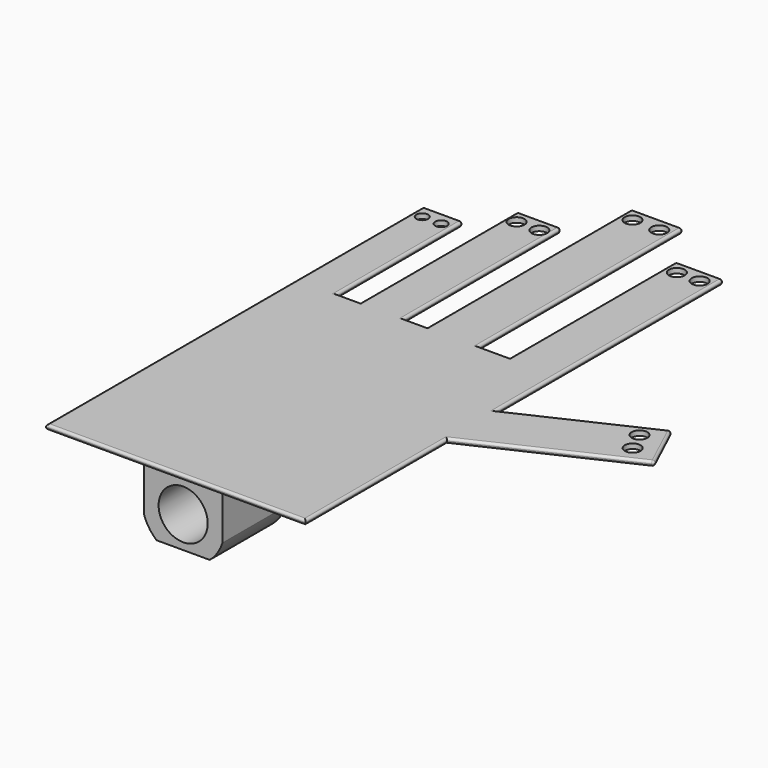
from build123d import *

# Parameters (mm, degrees)
F0_W          = 12.7
F0_H          = 50.8
F0_W_2        = 13.97
F0_H_2        = 63.5
F0_W_3        = 16.51
F0_H_3        = 82.55
F0_W_4        = 15.24
F0_H_4        = 67.123832345
F1_DEPTH      = 1.5875
F2_R          = 0.762
F3_R          = 0.762
F4_T1_DEPTH   = 87.63
F4_T3_DEPTH   = 153.543
F4_T5_DEPTH   = 66.361832345
F4_T7_DEPTH   = 50.038
F4_T9_DEPTH   = 10.16
F4_T11_DEPTH  = 7.62
F4_T13_DEPTH  = 81.788
F4_T15_DEPTH  = 62.738
F4_T17_DEPTH  = 7.62
F4_T19_DEPTH  = 0.0635
F4_T24_DEPTH  = 55.0115454207
F4_T29_DEPTH  = 61.0436683929
F4_T34_DEPTH  = 46.7205952588
F4_T39_DEPTH  = 93.015104553
F4_T44_DEPTH  = 55.0115454207
F4_T49_DEPTH  = 61.0436683929
F4_T54_DEPTH  = 46.7205952588
F4_T59_DEPTH  = 93.015104553
F4_T62_ANGLE  = 90
F4_T64_ANGLE  = 90
F4_T66_ANGLE  = 90
F4_T68_ANGLE  = 90
F4_T70_ANGLE  = 90
F4_T72_ANGLE  = 90
F4_T74_ANGLE  = 90
F4_T76_ANGLE  = 90
F4_T78_ANGLE  = 90
F4_T80_ANGLE  = 90
F4_T82_ANGLE  = 90
F4_T84_ANGLE  = 90
F4_T86_ANGLE  = 90
F4_T88_ANGLE  = 90
F4_T90_ANGLE  = 90
F4_T92_ANGLE  = 90
F4_T94_ANGLE  = 90
F4_T96_ANGLE  = 90
F4_T98_ANGLE  = 90
F4_T100_ANGLE = 90
F4_T105_DEPTH = 55.0115454207
F4_T109_DEPTH = 61.0436683929
F4_T116_DEPTH = 46.7205952588
F4_T120_DEPTH = 93.015104553
F4_T127_DEPTH = 68.266832345
F4_T131_DEPTH = 12.065
F4_T138_DEPTH = 51.943
F4_T142_DEPTH = 9.525
F4_T149_DEPTH = 12.065
F4_T153_DEPTH = 83.693
F4_T160_DEPTH = 9.525
F4_T164_DEPTH = 64.643
F4_T171_DEPTH = 83.693
F4_T175_DEPTH = 9.525
F4_T182_DEPTH = 64.643
F4_T186_DEPTH = 9.525
F4_T193_DEPTH = 55.0115454207
F4_T197_DEPTH = 61.0436683929
F4_T204_DEPTH = 46.7205952588
F4_T208_DEPTH = 93.015104553
F4_T215_DEPTH = 68.266832345
F4_T219_DEPTH = 12.065
F4_T226_DEPTH = 51.943
F4_T230_DEPTH = 9.525
F4_T237_DEPTH = 12.065
F4_T241_DEPTH = 83.693
F4_T248_DEPTH = 9.525
F4_T252_DEPTH = 64.643
F4_T259_DEPTH = 83.693
F4_T263_DEPTH = 9.525
F4_T270_DEPTH = 64.643
F4_T274_DEPTH = 9.525
F5_R          = 2.54
F5_R_2        = 1.905
F6_DEPTH      = 25.4
F7_W          = 25.4
F7_H          = 25.4
F8_DEPTH      = 20.32
F9_R          = 7.9375
F10_DEPTH     = 25.4
F12_DEPTH     = 25.4


# Not quite as in the source:
# - a fillet or chamfer that OpenCascade refuses, or shapes differently, is made with other operations: its cross-section is extruded or revolved along the edge and cut away or added


with BuildPart() as f1:
    # F0 (on Top) → F1 (new body)
    with BuildSketch(Plane.XY):
        Polygon((-47.5871736486, 71.2477097511), (-47.5871736486, -30.3522902489), (36.2328263514, -30.3522902489), (36.2328263514, 26.881378144), (36.2328263514, 46.4994375432), (36.2328263514, 71.2477097511), (20.9928263514, 71.2477097511), (10.8328263514, 71.2477097511), (-5.6771736486, 71.2477097511), (-13.2971736486, 71.2477097511), (-27.2671736486, 71.2477097511), (-34.8871736486, 71.2477097511), align=None)
        with Locations((-41.2371736486, 96.6477097511)):
            Rectangle(F0_W, F0_H)
        with Locations((-20.2821736486, 102.9977097511)):
            Rectangle(F0_W_2, F0_H_2)
        with Locations((2.5778263514, 112.5227097511)):
            Rectangle(F0_W_3, F0_H_3)
        with Locations((28.6128263514, 104.8096259236)):
            Rectangle(F0_W_4, F0_H_4)
        Polygon((36.2328263514, 46.4994375432), (36.2328263514, 26.881378144), (85.0543085426, 49.6472091722), (77.5401558489, 65.7613616258), align=None)
    extrude(amount=F1_DEPTH)

    # F2
    f2_edges = [f1.edges().sort_by_distance(p)[0] for p in [
        (-41.237174, 122.04771, 1.5875),
        (-20.282174, 134.74771, 1.5875),
        (2.577826, 153.79771, 1.5875),
        (28.612826, 138.371542, 1.5875),
        (81.297232, 57.704285, 1.5875),
    ]]
    fillet(f2_edges, radius=F2_R)

    # F3
    f3_edges = [f1.edges().sort_by_distance(p)[0] for p in [
        (81.297232, 57.704285, 0),
        (28.612826, 138.371542, 0),
        (2.577826, 153.79771, 0),
        (-20.282174, 134.74771, 0),
        (-41.237174, 122.04771, 0),
    ]]
    fillet(f3_edges, radius=F3_R)

    # F4: fillet of radius 0.762 on 70 edges, made by hand

    # F4_s2 → F4_t1 (cut)
    with BuildSketch(Plane.YZ.offset(-49.4921736486)):
        with BuildLine():
            ThreePointArc((-29.5902902489, 1.5875), (-30.1291056161, 1.3643153673), (-30.3522902489, 0.8255))
            Line((-30.3522902489, 0.8255), (-30.3522902489, 1.5875))
            Line((-30.3522902489, 1.5875), (-29.5902902489, 1.5875))
        make_face()
        with BuildLine():
            ThreePointArc((-29.5902902489, 0), (-30.1291056161, 0.2231846327), (-30.3522902489, 0.762))
            Line((-30.3522902489, 0.762), (-30.3522902489, 0))
            Line((-30.3522902489, 0), (-29.5902902489, 0))
        make_face()
    extrude(amount=F4_T1_DEPTH, mode=Mode.SUBTRACT)

    # F4_s4 → F4_t3 (cut)
    with BuildSketch(Plane.XZ.offset(-121.2857097511)):
        with BuildLine():
            ThreePointArc((-46.8251736486, 1.5875), (-47.3639890158, 1.3643153673), (-47.5871736486, 0.8255))
            Line((-47.5871736486, 0.8255), (-47.5871736486, 1.5875))
            Line((-47.5871736486, 1.5875), (-46.8251736486, 1.5875))
        make_face()
        with BuildLine():
            ThreePointArc((-46.8251736486, 0), (-47.3639890158, 0.2231846327), (-47.5871736486, 0.762))
            Line((-47.5871736486, 0.762), (-47.5871736486, 0))
            Line((-47.5871736486, 0), (-46.8251736486, 0))
        make_face()
    extrude(amount=F4_T3_DEPTH, mode=Mode.SUBTRACT)

    # F4_s6 → F4_t5 (cut)
    with BuildSketch(Plane.XZ.offset(-137.6095420961)):
        with BuildLine():
            ThreePointArc((21.7548263514, 1.5875), (21.2160109842, 1.3643153673), (20.9928263514, 0.8255))
            Line((20.9928263514, 0.8255), (20.9928263514, 1.5875))
            Line((20.9928263514, 1.5875), (21.7548263514, 1.5875))
        make_face()
        with BuildLine():
            ThreePointArc((21.7548263514, 0), (21.2160109842, 0.2231846327), (20.9928263514, 0.762))
            Line((20.9928263514, 0.762), (20.9928263514, 0))
            Line((20.9928263514, 0), (21.7548263514, 0))
        make_face()
    extrude(amount=F4_T5_DEPTH, mode=Mode.SUBTRACT)

    # F4_s8 → F4_t7 (cut)
    with BuildSketch(Plane.XZ.offset(-121.2857097511)):
        with BuildLine():
            ThreePointArc((-35.6491736486, 1.5875), (-35.1103582813, 1.3643153673), (-34.8871736486, 0.8255))
            Line((-34.8871736486, 0.8255), (-34.8871736486, 1.5875))
            Line((-34.8871736486, 1.5875), (-35.6491736486, 1.5875))
        make_face()
        with BuildLine():
            ThreePointArc((-35.6491736486, 0), (-35.1103582813, 0.2231846327), (-34.8871736486, 0.762))
            Line((-34.8871736486, 0.762), (-34.8871736486, 0))
            Line((-34.8871736486, 0), (-35.6491736486, 0))
        make_face()
    extrude(amount=F4_T7_DEPTH, mode=Mode.SUBTRACT)

    # F4_s10 → F4_t9 (cut)
    with BuildSketch(Plane.YZ.offset(10.8328263514)):
        with BuildLine():
            ThreePointArc((70.4857097511, 1.5875), (71.0245251184, 1.3643153673), (71.2477097511, 0.8255))
            Line((71.2477097511, 0.8255), (71.2477097511, 1.5875))
            Line((71.2477097511, 1.5875), (70.4857097511, 1.5875))
        make_face()
        with BuildLine():
            ThreePointArc((70.4857097511, 0), (71.0245251184, 0.2231846327), (71.2477097511, 0.762))
            Line((71.2477097511, 0.762), (71.2477097511, 0))
            Line((71.2477097511, 0), (70.4857097511, 0))
        make_face()
    extrude(amount=F4_T9_DEPTH, mode=Mode.SUBTRACT)

    # F4_s12 → F4_t11 (cut)
    with BuildSketch(Plane.YZ.offset(-34.8871736486)):
        with BuildLine():
            ThreePointArc((70.4857097511, 1.5875), (71.0245251184, 1.3643153673), (71.2477097511, 0.8255))
            Line((71.2477097511, 0.8255), (71.2477097511, 1.5875))
            Line((71.2477097511, 1.5875), (70.4857097511, 1.5875))
        make_face()
        with BuildLine():
            ThreePointArc((70.4857097511, 0), (71.0245251184, 0.2231846327), (71.2477097511, 0.762))
            Line((71.2477097511, 0.762), (71.2477097511, 0))
            Line((71.2477097511, 0), (70.4857097511, 0))
        make_face()
    extrude(amount=F4_T11_DEPTH, mode=Mode.SUBTRACT)

    # F4_s14 → F4_t13 (cut)
    with BuildSketch(Plane.XZ.offset(-153.0357097511)):
        with BuildLine():
            ThreePointArc((10.0708263514, 1.5875), (10.6096417187, 1.3643153673), (10.8328263514, 0.8255))
            Line((10.8328263514, 0.8255), (10.8328263514, 1.5875))
            Line((10.8328263514, 1.5875), (10.0708263514, 1.5875))
        make_face()
        with BuildLine():
            ThreePointArc((-4.9151736486, 1.5875), (-5.4539890158, 1.3643153673), (-5.6771736486, 0.8255))
            Line((-5.6771736486, 0.8255), (-5.6771736486, 1.5875))
            Line((-5.6771736486, 1.5875), (-4.9151736486, 1.5875))
        make_face()
        with BuildLine():
            ThreePointArc((10.0708263514, 0), (10.6096417187, 0.2231846327), (10.8328263514, 0.762))
            Line((10.8328263514, 0.762), (10.8328263514, 0))
            Line((10.8328263514, 0), (10.0708263514, 0))
        make_face()
        with BuildLine():
            ThreePointArc((-4.9151736486, 0), (-5.4539890158, 0.2231846327), (-5.6771736486, 0.762))
            Line((-5.6771736486, 0.762), (-5.6771736486, 0))
            Line((-5.6771736486, 0), (-4.9151736486, 0))
        make_face()
    extrude(amount=F4_T13_DEPTH, mode=Mode.SUBTRACT)

    # F4_s16 → F4_t15 (cut)
    with BuildSketch(Plane.XZ.offset(-133.9857097511)):
        with BuildLine():
            ThreePointArc((-26.5051736486, 1.5875), (-27.0439890158, 1.3643153673), (-27.2671736486, 0.8255))
            Line((-27.2671736486, 0.8255), (-27.2671736486, 1.5875))
            Line((-27.2671736486, 1.5875), (-26.5051736486, 1.5875))
        make_face()
        with BuildLine():
            ThreePointArc((-14.0591736486, 1.5875), (-13.5203582813, 1.3643153673), (-13.2971736486, 0.8255))
            Line((-13.2971736486, 0.8255), (-13.2971736486, 1.5875))
            Line((-13.2971736486, 1.5875), (-14.0591736486, 1.5875))
        make_face()
        with BuildLine():
            ThreePointArc((-26.5051736486, 0), (-27.0439890158, 0.2231846327), (-27.2671736486, 0.762))
            Line((-27.2671736486, 0.762), (-27.2671736486, 0))
            Line((-27.2671736486, 0), (-26.5051736486, 0))
        make_face()
        with BuildLine():
            ThreePointArc((-14.0591736486, 0), (-13.5203582813, 0.2231846327), (-13.2971736486, 0.762))
            Line((-13.2971736486, 0.762), (-13.2971736486, 0))
            Line((-13.2971736486, 0), (-14.0591736486, 0))
        make_face()
    extrude(amount=F4_T15_DEPTH, mode=Mode.SUBTRACT)

    # F4_s18 → F4_t17 (cut)
    with BuildSketch(Plane.YZ.offset(-13.2971736486)):
        with BuildLine():
            ThreePointArc((70.4857097511, 1.5875), (71.0245251184, 1.3643153673), (71.2477097511, 0.8255))
            Line((71.2477097511, 0.8255), (71.2477097511, 1.5875))
            Line((71.2477097511, 1.5875), (70.4857097511, 1.5875))
        make_face()
        with BuildLine():
            ThreePointArc((70.4857097511, 0), (71.0245251184, 0.2231846327), (71.2477097511, 0.762))
            Line((71.2477097511, 0.762), (71.2477097511, 0))
            Line((71.2477097511, 0), (70.4857097511, 0))
        make_face()
    extrude(amount=F4_T17_DEPTH, mode=Mode.SUBTRACT)

    # F4_s20 → F4_t19 (cut)
    with BuildSketch(Plane.XY.offset(0.762)):
        with BuildLine():
            ThreePointArc((84.3637020089, 49.3251740568), (84.7577126705, 49.7551612413), (84.7322734272, 50.337815706))
            Line((84.7322734272, 50.337815706), (85.0543085426, 49.6472091722))
            Line((85.0543085426, 49.6472091722), (84.3637020089, 49.3251740568))
        make_face()
        with BuildLine():
            ThreePointArc((77.8621909643, 65.070755092), (77.4322037798, 65.4647657536), (76.8495493151, 65.4393265103))
            Line((76.8495493151, 65.4393265103), (77.5401558489, 65.7613616258))
            Line((77.5401558489, 65.7613616258), (77.8621909643, 65.070755092))
        make_face()
        with BuildLine():
            ThreePointArc((36.2328263514, 137.6095420961), (36.0096417187, 138.1483574634), (35.4708263514, 138.3715420961))
            Line((35.4708263514, 138.3715420961), (36.2328263514, 138.3715420961))
            Line((36.2328263514, 138.3715420961), (36.2328263514, 137.6095420961))
        make_face()
        with BuildLine():
            ThreePointArc((-47.5871736486, 121.2857097511), (-47.3639890158, 121.8245251184), (-46.8251736486, 122.0477097511))
            Line((-46.8251736486, 122.0477097511), (-47.5871736486, 122.0477097511))
            Line((-47.5871736486, 122.0477097511), (-47.5871736486, 121.2857097511))
        make_face()
        with BuildLine():
            ThreePointArc((20.9928263514, 137.6095420961), (21.2160109842, 138.1483574634), (21.7548263514, 138.3715420961))
            Line((21.7548263514, 138.3715420961), (20.9928263514, 138.3715420961))
            Line((20.9928263514, 138.3715420961), (20.9928263514, 137.6095420961))
        make_face()
        with BuildLine():
            ThreePointArc((-34.8871736486, 121.2857097511), (-35.1103582813, 121.8245251184), (-35.6491736486, 122.0477097511))
            Line((-35.6491736486, 122.0477097511), (-34.8871736486, 122.0477097511))
            Line((-34.8871736486, 122.0477097511), (-34.8871736486, 121.2857097511))
        make_face()
        with BuildLine():
            ThreePointArc((10.8328263514, 153.0357097511), (10.6096417187, 153.5745251184), (10.0708263514, 153.7977097511))
            Line((10.0708263514, 153.7977097511), (10.8328263514, 153.7977097511))
            Line((10.8328263514, 153.7977097511), (10.8328263514, 153.0357097511))
        make_face()
        with BuildLine():
            ThreePointArc((-27.2671736486, 133.9857097511), (-27.0439890158, 134.5245251184), (-26.5051736486, 134.7477097511))
            Line((-26.5051736486, 134.7477097511), (-27.2671736486, 134.7477097511))
            Line((-27.2671736486, 134.7477097511), (-27.2671736486, 133.9857097511))
        make_face()
        with BuildLine():
            ThreePointArc((-5.6771736486, 153.0357097511), (-5.4539890158, 153.5745251184), (-4.9151736486, 153.7977097511))
            Line((-4.9151736486, 153.7977097511), (-5.6771736486, 153.7977097511))
            Line((-5.6771736486, 153.7977097511), (-5.6771736486, 153.0357097511))
        make_face()
        with BuildLine():
            ThreePointArc((-13.2971736486, 133.9857097511), (-13.5203582813, 134.5245251184), (-14.0591736486, 134.7477097511))
            Line((-14.0591736486, 134.7477097511), (-13.2971736486, 134.7477097511))
            Line((-13.2971736486, 134.7477097511), (-13.2971736486, 133.9857097511))
        make_face()
    extrude(amount=F4_T19_DEPTH, mode=Mode.SUBTRACT)


with BuildPart() as f4_tool22:
    # F4_s23 → F4_t24 (new body)
    with BuildSketch(Plane(origin=(38.331067938, 17.8740705248, 0), x_dir=(0, 0, 1), z_dir=(0.906307787, 0.4226182617, 0))):
        with BuildLine():
            ThreePointArc((0.8255, -9.0501482476), (1.3643153673, -9.2733328803), (1.5875, -9.8121482476))
            Line((1.5875, -9.8121482476), (1.5875, -9.0501482476))
            Line((1.5875, -9.0501482476), (0.8255, -9.0501482476))
        make_face()
    extrude(amount=F4_T24_DEPTH)

    split(bisect_by=Plane.YZ.offset(36.2328263514), keep=Keep.TOP)


with BuildPart() as f1_1:
    add(f1.part)

    # F4_t21: cut F4_tool22
    add(f4_tool22.part, mode=Mode.SUBTRACT)


with BuildPart() as f4_tool27:
    # F4_s28 → F4_t29 (new body)
    with BuildSketch(Plane.XZ.offset(32.2572902489)):
        with BuildLine():
            ThreePointArc((35.4708263514, 1.5875), (36.0096417187, 1.3643153673), (36.2328263514, 0.8255))
            Line((36.2328263514, 0.8255), (36.2328263514, 1.5875))
            Line((36.2328263514, 1.5875), (35.4708263514, 1.5875))
        make_face()
    extrude(amount=-F4_T29_DEPTH)

    split(bisect_by=Plane(origin=(-3.8247579209, 8.2022198306, 0), x_dir=(0, 0, 1), z_dir=(0.4226182617, -0.906307787, 0)), keep=Keep.TOP)


with BuildPart() as f1_2:
    add(f1_1.part)

    # F4_t26: cut F4_tool27
    add(f4_tool27.part, mode=Mode.SUBTRACT)


with BuildPart() as f4_tool32:
    # F4_s33 → F4_t34 (new body)
    with BuildSketch(Plane(origin=(88.1884599298, 41.1229542262, 0), x_dir=(0, 0, 1), z_dir=(-0.906307787, -0.4226182617, 0))):
        with BuildLine():
            ThreePointArc((1.5875, 26.0681482476), (1.3643153673, 26.6069636149), (0.8255, 26.8301482476))
            Line((0.8255, 26.8301482476), (1.5875, 26.8301482476))
            Line((1.5875, 26.8301482476), (1.5875, 26.0681482476))
        make_face()
    extrude(amount=F4_T34_DEPTH)

    split(bisect_by=Plane.YZ.offset(36.2328263514), keep=Keep.TOP)


with BuildPart() as f1_3:
    add(f1_2.part)

    # F4_t31: cut F4_tool32
    add(f4_tool32.part, mode=Mode.SUBTRACT)


with BuildPart() as f4_tool37:
    # F4_s38 → F4_t39 (new body)
    with BuildSketch(Plane.XZ.offset(-44.5944375432)):
        with BuildLine():
            ThreePointArc((35.4708263514, 1.5875), (36.0096417187, 1.3643153673), (36.2328263514, 0.8255))
            Line((36.2328263514, 0.8255), (36.2328263514, 1.5875))
            Line((36.2328263514, 1.5875), (35.4708263514, 1.5875))
        make_face()
    extrude(amount=-F4_T39_DEPTH)

    split(bisect_by=Plane(origin=(-11.3389106146, 24.3163722842, 0), x_dir=(0, 0, 1), z_dir=(-0.4226182617, 0.906307787, 0)), keep=Keep.TOP)


with BuildPart() as f1_4:
    add(f1_3.part)

    # F4_t36: cut F4_tool37
    add(f4_tool37.part, mode=Mode.SUBTRACT)


with BuildPart() as f4_tool42:
    # F4_s43 → F4_t44 (new body)
    with BuildSketch(Plane(origin=(38.331067938, 17.8740705248, 0), x_dir=(0, 0, 1), z_dir=(0.906307787, 0.4226182617, 0))):
        with BuildLine():
            ThreePointArc((0.762, -9.0501482476), (0.2231846327, -9.2733328803), (0, -9.8121482476))
            Line((0, -9.8121482476), (0, -9.0501482476))
            Line((0, -9.0501482476), (0.762, -9.0501482476))
        make_face()
    extrude(amount=F4_T44_DEPTH)

    split(bisect_by=Plane.YZ.offset(36.2328263514), keep=Keep.TOP)


with BuildPart() as f1_5:
    add(f1_4.part)

    # F4_t41: cut F4_tool42
    add(f4_tool42.part, mode=Mode.SUBTRACT)


with BuildPart() as f4_tool47:
    # F4_s48 → F4_t49 (new body)
    with BuildSketch(Plane.XZ.offset(32.2572902489)):
        with BuildLine():
            ThreePointArc((35.4708263514, 0), (36.0096417187, 0.2231846327), (36.2328263514, 0.762))
            Line((36.2328263514, 0.762), (36.2328263514, 0))
            Line((36.2328263514, 0), (35.4708263514, 0))
        make_face()
    extrude(amount=-F4_T49_DEPTH)

    split(bisect_by=Plane(origin=(-3.8247579209, 8.2022198306, 0), x_dir=(0, 0, 1), z_dir=(0.4226182617, -0.906307787, 0)), keep=Keep.TOP)


with BuildPart() as f1_6:
    add(f1_5.part)

    # F4_t46: cut F4_tool47
    add(f4_tool47.part, mode=Mode.SUBTRACT)


with BuildPart() as f4_tool52:
    # F4_s53 → F4_t54 (new body)
    with BuildSketch(Plane(origin=(88.1884599298, 41.1229542262, 0), x_dir=(0, 0, 1), z_dir=(-0.906307787, -0.4226182617, 0))):
        with BuildLine():
            ThreePointArc((0, 26.0681482476), (0.2231846327, 26.6069636149), (0.762, 26.8301482476))
            Line((0.762, 26.8301482476), (0, 26.8301482476))
            Line((0, 26.8301482476), (0, 26.0681482476))
        make_face()
    extrude(amount=F4_T54_DEPTH)

    split(bisect_by=Plane.YZ.offset(36.2328263514), keep=Keep.TOP)


with BuildPart() as f1_7:
    add(f1_6.part)

    # F4_t51: cut F4_tool52
    add(f4_tool52.part, mode=Mode.SUBTRACT)


with BuildPart() as f4_tool57:
    # F4_s58 → F4_t59 (new body)
    with BuildSketch(Plane.XZ.offset(-44.5944375432)):
        with BuildLine():
            ThreePointArc((35.4708263514, 0), (36.0096417187, 0.2231846327), (36.2328263514, 0.762))
            Line((36.2328263514, 0.762), (36.2328263514, 0))
            Line((36.2328263514, 0), (35.4708263514, 0))
        make_face()
    extrude(amount=-F4_T59_DEPTH)

    split(bisect_by=Plane(origin=(-11.3389106146, 24.3163722842, 0), x_dir=(0, 0, 1), z_dir=(-0.4226182617, 0.906307787, 0)), keep=Keep.TOP)


with BuildPart() as f1_8:
    add(f1_7.part)

    # F4_t56: cut F4_tool57
    add(f4_tool57.part, mode=Mode.SUBTRACT)

    # F4_s61 → F4_t62 (revolve, cut)
    with BuildSketch(Plane.XY.offset(0.762)):
        with BuildLine():
            ThreePointArc((84.3637020089, 49.3251740568), (84.7577126705, 49.7551612413), (84.7322734272, 50.337815706))
            Line((84.7322734272, 50.337815706), (85.0543085426, 49.6472091722))
            Line((85.0543085426, 49.6472091722), (84.3637020089, 49.3251740568))
        make_face()
    revolve(axis=Axis((84.3637020089, 49.3251740568, 0.762), (-0.4226182617, 0.906307787, 0)), revolution_arc=F4_T62_ANGLE, mode=Mode.SUBTRACT)

    # F4_s63 → F4_t64 (revolve, cut)
    with BuildSketch(Plane.XY.offset(0.8255)):
        with BuildLine():
            ThreePointArc((84.3637020089, 49.3251740568), (84.7577126705, 49.7551612413), (84.7322734272, 50.337815706))
            Line((84.7322734272, 50.337815706), (85.0543085426, 49.6472091722))
            Line((85.0543085426, 49.6472091722), (84.3637020089, 49.3251740568))
        make_face()
    revolve(axis=Axis((84.3637020089, 49.3251740568, 0.8255), (0.4226182617, -0.906307787, 0)), revolution_arc=F4_T64_ANGLE, mode=Mode.SUBTRACT)

    # F4_s65 → F4_t66 (revolve, cut)
    with BuildSketch(Plane.XY.offset(0.762)):
        with BuildLine():
            ThreePointArc((77.8621909643, 65.070755092), (77.4322037798, 65.4647657536), (76.8495493151, 65.4393265103))
            Line((76.8495493151, 65.4393265103), (77.5401558489, 65.7613616258))
            Line((77.5401558489, 65.7613616258), (77.8621909643, 65.070755092))
        make_face()
    revolve(axis=Axis((76.8495493151, 65.4393265103, 0.762), (-0.4226182617, 0.906307787, 0)), revolution_arc=F4_T66_ANGLE, mode=Mode.SUBTRACT)

    # F4_s67 → F4_t68 (revolve, cut)
    with BuildSketch(Plane.XY.offset(0.8255)):
        with BuildLine():
            ThreePointArc((77.8621909643, 65.070755092), (77.4322037798, 65.4647657536), (76.8495493151, 65.4393265103))
            Line((76.8495493151, 65.4393265103), (77.5401558489, 65.7613616258))
            Line((77.5401558489, 65.7613616258), (77.8621909643, 65.070755092))
        make_face()
    revolve(axis=Axis((76.8495493151, 65.4393265103, 0.8255), (0.4226182617, -0.906307787, 0)), revolution_arc=F4_T68_ANGLE, mode=Mode.SUBTRACT)

    # F4_s69 → F4_t70 (revolve, cut)
    with BuildSketch(Plane.XZ.offset(-137.6095420961)):
        with BuildLine():
            ThreePointArc((36.2328263514, 0.762), (36.0096417187, 0.2231846327), (35.4708263514, 0))
            Line((35.4708263514, 0), (36.2328263514, 0))
            Line((36.2328263514, 0), (36.2328263514, 0.762))
        make_face()
    revolve(axis=Axis((36.2328263514, 137.6095420961, 0.762), (1, 0, 0)), revolution_arc=F4_T70_ANGLE, mode=Mode.SUBTRACT)

    # F4_s71 → F4_t72 (revolve, cut)
    with BuildSketch(Plane.XY.offset(0.8255)):
        with BuildLine():
            ThreePointArc((36.2328263514, 137.6095420961), (36.0096417187, 138.1483574634), (35.4708263514, 138.3715420961))
            Line((35.4708263514, 138.3715420961), (36.2328263514, 138.3715420961))
            Line((36.2328263514, 138.3715420961), (36.2328263514, 137.6095420961))
        make_face()
    revolve(axis=Axis((36.2328263514, 137.6095420961, 0.8255), (1, 0, 0)), revolution_arc=F4_T72_ANGLE, mode=Mode.SUBTRACT)

    # F4_s73 → F4_t74 (revolve, cut)
    with BuildSketch(Plane.XZ.offset(-121.2857097511)):
        with BuildLine():
            ThreePointArc((-47.5871736486, 0.762), (-47.3639890158, 0.2231846327), (-46.8251736486, 0))
            Line((-46.8251736486, 0), (-47.5871736486, 0))
            Line((-47.5871736486, 0), (-47.5871736486, 0.762))
        make_face()
    revolve(axis=Axis((-47.5871736486, 121.2857097511, 0.762), (1, 0, 0)), revolution_arc=F4_T74_ANGLE, mode=Mode.SUBTRACT)

    # F4_s75 → F4_t76 (revolve, cut)
    with BuildSketch(Plane.XY.offset(0.8255)):
        with BuildLine():
            ThreePointArc((-47.5871736486, 121.2857097511), (-47.3639890158, 121.8245251184), (-46.8251736486, 122.0477097511))
            Line((-46.8251736486, 122.0477097511), (-47.5871736486, 122.0477097511))
            Line((-47.5871736486, 122.0477097511), (-47.5871736486, 121.2857097511))
        make_face()
    revolve(axis=Axis((-47.5871736486, 121.2857097511, 0.8255), (1, 0, 0)), revolution_arc=F4_T76_ANGLE, mode=Mode.SUBTRACT)

    # F4_s77 → F4_t78 (revolve, cut)
    with BuildSketch(Plane.XZ.offset(-137.6095420961)):
        with BuildLine():
            ThreePointArc((21.7548263514, 0), (21.2160109842, 0.2231846327), (20.9928263514, 0.762))
            Line((20.9928263514, 0.762), (20.9928263514, 0))
            Line((20.9928263514, 0), (21.7548263514, 0))
        make_face()
    revolve(axis=Axis((20.9928263514, 137.6095420961, 0.762), (1, 0, 0)), revolution_arc=F4_T78_ANGLE, mode=Mode.SUBTRACT)

    # F4_s79 → F4_t80 (revolve, cut)
    with BuildSketch(Plane.XZ.offset(-121.2857097511)):
        with BuildLine():
            ThreePointArc((-35.6491736486, 0), (-35.1103582813, 0.2231846327), (-34.8871736486, 0.762))
            Line((-34.8871736486, 0.762), (-34.8871736486, 0))
            Line((-34.8871736486, 0), (-35.6491736486, 0))
        make_face()
    revolve(axis=Axis((-34.8871736486, 121.2857097511, 0.762), (1, 0, 0)), revolution_arc=F4_T80_ANGLE, mode=Mode.SUBTRACT)

    # F4_s81 → F4_t82 (revolve, cut)
    with BuildSketch(Plane.XY.offset(0.8255)):
        with BuildLine():
            ThreePointArc((20.9928263514, 137.6095420961), (21.2160109842, 138.1483574634), (21.7548263514, 138.3715420961))
            Line((21.7548263514, 138.3715420961), (20.9928263514, 138.3715420961))
            Line((20.9928263514, 138.3715420961), (20.9928263514, 137.6095420961))
        make_face()
    revolve(axis=Axis((20.9928263514, 137.6095420961, 0.8255), (1, 0, 0)), revolution_arc=F4_T82_ANGLE, mode=Mode.SUBTRACT)

    # F4_s83 → F4_t84 (revolve, cut)
    with BuildSketch(Plane.XY.offset(0.8255)):
        with BuildLine():
            ThreePointArc((-34.8871736486, 121.2857097511), (-35.1103582813, 121.8245251184), (-35.6491736486, 122.0477097511))
            Line((-35.6491736486, 122.0477097511), (-34.8871736486, 122.0477097511))
            Line((-34.8871736486, 122.0477097511), (-34.8871736486, 121.2857097511))
        make_face()
    revolve(axis=Axis((-34.8871736486, 121.2857097511, 0.8255), (1, 0, 0)), revolution_arc=F4_T84_ANGLE, mode=Mode.SUBTRACT)

    # F4_s85 → F4_t86 (revolve, cut)
    with BuildSketch(Plane.XZ.offset(-153.0357097511)):
        with BuildLine():
            ThreePointArc((10.8328263514, 0.762), (10.6096417187, 0.2231846327), (10.0708263514, 0))
            Line((10.0708263514, 0), (10.8328263514, 0))
            Line((10.8328263514, 0), (10.8328263514, 0.762))
        make_face()
    revolve(axis=Axis((10.8328263514, 153.0357097511, 0.762), (1, 0, 0)), revolution_arc=F4_T86_ANGLE, mode=Mode.SUBTRACT)

    # F4_s87 → F4_t88 (revolve, cut)
    with BuildSketch(Plane.XY.offset(0.8255)):
        with BuildLine():
            ThreePointArc((10.8328263514, 153.0357097511), (10.6096417187, 153.5745251184), (10.0708263514, 153.7977097511))
            Line((10.0708263514, 153.7977097511), (10.8328263514, 153.7977097511))
            Line((10.8328263514, 153.7977097511), (10.8328263514, 153.0357097511))
        make_face()
    revolve(axis=Axis((10.8328263514, 153.0357097511, 0.8255), (1, 0, 0)), revolution_arc=F4_T88_ANGLE, mode=Mode.SUBTRACT)

    # F4_s89 → F4_t90 (revolve, cut)
    with BuildSketch(Plane.XZ.offset(-133.9857097511)):
        with BuildLine():
            ThreePointArc((-27.2671736486, 0.762), (-27.0439890158, 0.2231846327), (-26.5051736486, 0))
            Line((-26.5051736486, 0), (-27.2671736486, 0))
            Line((-27.2671736486, 0), (-27.2671736486, 0.762))
        make_face()
    revolve(axis=Axis((-27.2671736486, 133.9857097511, 0.762), (1, 0, 0)), revolution_arc=F4_T90_ANGLE, mode=Mode.SUBTRACT)

    # F4_s91 → F4_t92 (revolve, cut)
    with BuildSketch(Plane.XY.offset(0.8255)):
        with BuildLine():
            ThreePointArc((-27.2671736486, 133.9857097511), (-27.0439890158, 134.5245251184), (-26.5051736486, 134.7477097511))
            Line((-26.5051736486, 134.7477097511), (-27.2671736486, 134.7477097511))
            Line((-27.2671736486, 134.7477097511), (-27.2671736486, 133.9857097511))
        make_face()
    revolve(axis=Axis((-27.2671736486, 133.9857097511, 0.8255), (1, 0, 0)), revolution_arc=F4_T92_ANGLE, mode=Mode.SUBTRACT)

    # F4_s93 → F4_t94 (revolve, cut)
    with BuildSketch(Plane.XZ.offset(-153.0357097511)):
        with BuildLine():
            ThreePointArc((-4.9151736486, 0), (-5.4539890158, 0.2231846327), (-5.6771736486, 0.762))
            Line((-5.6771736486, 0.762), (-5.6771736486, 0))
            Line((-5.6771736486, 0), (-4.9151736486, 0))
        make_face()
    revolve(axis=Axis((-5.6771736486, 153.0357097511, 0.762), (1, 0, 0)), revolution_arc=F4_T94_ANGLE, mode=Mode.SUBTRACT)

    # F4_s95 → F4_t96 (revolve, cut)
    with BuildSketch(Plane.XZ.offset(-133.9857097511)):
        with BuildLine():
            ThreePointArc((-14.0591736486, 0), (-13.5203582813, 0.2231846327), (-13.2971736486, 0.762))
            Line((-13.2971736486, 0.762), (-13.2971736486, 0))
            Line((-13.2971736486, 0), (-14.0591736486, 0))
        make_face()
    revolve(axis=Axis((-13.2971736486, 133.9857097511, 0.762), (1, 0, 0)), revolution_arc=F4_T96_ANGLE, mode=Mode.SUBTRACT)

    # F4_s97 → F4_t98 (revolve, cut)
    with BuildSketch(Plane.XY.offset(0.8255)):
        with BuildLine():
            ThreePointArc((-5.6771736486, 153.0357097511), (-5.4539890158, 153.5745251184), (-4.9151736486, 153.7977097511))
            Line((-4.9151736486, 153.7977097511), (-5.6771736486, 153.7977097511))
            Line((-5.6771736486, 153.7977097511), (-5.6771736486, 153.0357097511))
        make_face()
    revolve(axis=Axis((-5.6771736486, 153.0357097511, 0.8255), (1, 0, 0)), revolution_arc=F4_T98_ANGLE, mode=Mode.SUBTRACT)

    # F4_s99 → F4_t100 (revolve, cut)
    with BuildSketch(Plane.XY.offset(0.8255)):
        with BuildLine():
            ThreePointArc((-13.2971736486, 133.9857097511), (-13.5203582813, 134.5245251184), (-14.0591736486, 134.7477097511))
            Line((-14.0591736486, 134.7477097511), (-13.2971736486, 134.7477097511))
            Line((-13.2971736486, 134.7477097511), (-13.2971736486, 133.9857097511))
        make_face()
    revolve(axis=Axis((-13.2971736486, 133.9857097511, 0.8255), (1, 0, 0)), revolution_arc=F4_T100_ANGLE, mode=Mode.SUBTRACT)


with BuildPart() as f4_tool103:
    # F4_s104 → F4_t105 (new body)
    with BuildSketch(Plane(origin=(38.331067938, 17.8740705248, 0), x_dir=(0, 0, 1), z_dir=(0.906307787, 0.4226182617, 0))):
        with BuildLine():
            ThreePointArc((0.8255, -9.0501482476), (1.3643153673, -9.2733328803), (1.5875, -9.8121482476))
            Line((1.5875, -9.8121482476), (1.5875, -9.0501482476))
            Line((1.5875, -9.0501482476), (0.8255, -9.0501482476))
        make_face()
    extrude(amount=F4_T105_DEPTH)

    split(bisect_by=Plane.YZ.offset(36.2328263514), keep=Keep.BOTTOM)


with BuildPart() as f4_tool107:
    # F4_s108 → F4_t109 (new body)
    with BuildSketch(Plane.XZ.offset(32.2572902489)):
        with BuildLine():
            ThreePointArc((35.4708263514, 1.5875), (36.0096417187, 1.3643153673), (36.2328263514, 0.8255))
            Line((36.2328263514, 0.8255), (36.2328263514, 1.5875))
            Line((36.2328263514, 1.5875), (35.4708263514, 1.5875))
        make_face()
    extrude(amount=-F4_T109_DEPTH)

    split(bisect_by=Plane(origin=(-3.8247579209, 8.2022198306, 0), x_dir=(0, 0, 1), z_dir=(-0.4226182617, 0.906307787, 0)), keep=Keep.TOP)


with BuildPart() as f4_tool103_1:
    add(f4_tool103.part)

    # F4_t111: intersect F4_tool107
    add(f4_tool107.part, mode=Mode.INTERSECT)


with BuildPart() as f1_9:
    add(f1_8.part)

    # F4_t101: cut F4_tool103
    add(f4_tool103_1.part, mode=Mode.SUBTRACT)


with BuildPart() as f4_tool114:
    # F4_s115 → F4_t116 (new body)
    with BuildSketch(Plane(origin=(88.1884599298, 41.1229542262, 0), x_dir=(0, 0, 1), z_dir=(-0.906307787, -0.4226182617, 0))):
        with BuildLine():
            ThreePointArc((1.5875, 26.0681482476), (1.3643153673, 26.6069636149), (0.8255, 26.8301482476))
            Line((0.8255, 26.8301482476), (1.5875, 26.8301482476))
            Line((1.5875, 26.8301482476), (1.5875, 26.0681482476))
        make_face()
    extrude(amount=F4_T116_DEPTH)

    split(bisect_by=Plane.YZ.offset(36.2328263514), keep=Keep.BOTTOM)


with BuildPart() as f4_tool118:
    # F4_s119 → F4_t120 (new body)
    with BuildSketch(Plane.XZ.offset(-44.5944375432)):
        with BuildLine():
            ThreePointArc((35.4708263514, 1.5875), (36.0096417187, 1.3643153673), (36.2328263514, 0.8255))
            Line((36.2328263514, 0.8255), (36.2328263514, 1.5875))
            Line((36.2328263514, 1.5875), (35.4708263514, 1.5875))
        make_face()
    extrude(amount=-F4_T120_DEPTH)

    split(bisect_by=Plane(origin=(-11.3389106146, 24.3163722842, 0), x_dir=(0, 0, 1), z_dir=(0.4226182617, -0.906307787, 0)), keep=Keep.TOP)


with BuildPart() as f4_tool114_1:
    add(f4_tool114.part)

    # F4_t122: intersect F4_tool118
    add(f4_tool118.part, mode=Mode.INTERSECT)


with BuildPart() as f1_10:
    add(f1_9.part)

    # F4_t112: cut F4_tool114
    add(f4_tool114_1.part, mode=Mode.SUBTRACT)


with BuildPart() as f4_tool125:
    # F4_s126 → F4_t127 (new body)
    with BuildSketch(Plane.XZ.offset(-137.6095420961)):
        with BuildLine():
            ThreePointArc((21.7548263514, 1.5875), (21.2160109842, 1.3643153673), (20.9928263514, 0.8255))
            Line((20.9928263514, 0.8255), (20.9928263514, 1.5875))
            Line((20.9928263514, 1.5875), (21.7548263514, 1.5875))
        make_face()
    extrude(amount=F4_T127_DEPTH)

    split(bisect_by=Plane.XZ.offset(-71.2477097511), keep=Keep.TOP)


with BuildPart() as f4_tool129:
    # F4_s130 → F4_t131 (new body)
    with BuildSketch(Plane.YZ.offset(22.8978263514)):
        with BuildLine():
            ThreePointArc((70.4857097511, 1.5875), (71.0245251184, 1.3643153673), (71.2477097511, 0.8255))
            Line((71.2477097511, 0.8255), (71.2477097511, 1.5875))
            Line((71.2477097511, 1.5875), (70.4857097511, 1.5875))
        make_face()
    extrude(amount=-F4_T131_DEPTH)

    split(bisect_by=Plane.YZ.offset(20.9928263514), keep=Keep.TOP)


with BuildPart() as f4_tool125_1:
    add(f4_tool125.part)

    # F4_t133: intersect F4_tool129
    add(f4_tool129.part, mode=Mode.INTERSECT)


with BuildPart() as f1_11:
    add(f1_10.part)

    # F4_t123: cut F4_tool125
    add(f4_tool125_1.part, mode=Mode.SUBTRACT)


with BuildPart() as f4_tool136:
    # F4_s137 → F4_t138 (new body)
    with BuildSketch(Plane.XZ.offset(-69.3427097511)):
        with BuildLine():
            ThreePointArc((-35.6491736486, 1.5875), (-35.1103582813, 1.3643153673), (-34.8871736486, 0.8255))
            Line((-34.8871736486, 0.8255), (-34.8871736486, 1.5875))
            Line((-34.8871736486, 1.5875), (-35.6491736486, 1.5875))
        make_face()
    extrude(amount=-F4_T138_DEPTH)

    split(bisect_by=Plane.XZ.offset(-71.2477097511), keep=Keep.TOP)


with BuildPart() as f4_tool140:
    # F4_s141 → F4_t142 (new body)
    with BuildSketch(Plane.YZ.offset(-27.2671736486)):
        with BuildLine():
            ThreePointArc((70.4857097511, 1.5875), (71.0245251184, 1.3643153673), (71.2477097511, 0.8255))
            Line((71.2477097511, 0.8255), (71.2477097511, 1.5875))
            Line((71.2477097511, 1.5875), (70.4857097511, 1.5875))
        make_face()
    extrude(amount=-F4_T142_DEPTH)

    split(bisect_by=Plane.YZ.offset(-34.8871736486), keep=Keep.BOTTOM)


with BuildPart() as f4_tool136_1:
    add(f4_tool136.part)

    # F4_t144: intersect F4_tool140
    add(f4_tool140.part, mode=Mode.INTERSECT)


with BuildPart() as f1_12:
    add(f1_11.part)

    # F4_t134: cut F4_tool136
    add(f4_tool136_1.part, mode=Mode.SUBTRACT)


with BuildPart() as f4_tool147:
    # F4_s148 → F4_t149 (new body)
    with BuildSketch(Plane.YZ.offset(20.9928263514)):
        with BuildLine():
            ThreePointArc((70.4857097511, 1.5875), (71.0245251184, 1.3643153673), (71.2477097511, 0.8255))
            Line((71.2477097511, 0.8255), (71.2477097511, 1.5875))
            Line((71.2477097511, 1.5875), (70.4857097511, 1.5875))
        make_face()
    extrude(amount=-F4_T149_DEPTH)

    split(bisect_by=Plane.YZ.offset(10.8328263514), keep=Keep.BOTTOM)


with BuildPart() as f4_tool151:
    # F4_s152 → F4_t153 (new body)
    with BuildSketch(Plane.XZ.offset(-69.3427097511)):
        with BuildLine():
            ThreePointArc((10.0708263514, 1.5875), (10.6096417187, 1.3643153673), (10.8328263514, 0.8255))
            Line((10.8328263514, 0.8255), (10.8328263514, 1.5875))
            Line((10.8328263514, 1.5875), (10.0708263514, 1.5875))
        make_face()
    extrude(amount=-F4_T153_DEPTH)

    split(bisect_by=Plane.XZ.offset(-71.2477097511), keep=Keep.TOP)


with BuildPart() as f4_tool147_1:
    add(f4_tool147.part)

    # F4_t155: intersect F4_tool151
    add(f4_tool151.part, mode=Mode.INTERSECT)


with BuildPart() as f1_13:
    add(f1_12.part)

    # F4_t145: cut F4_tool147
    add(f4_tool147_1.part, mode=Mode.SUBTRACT)


with BuildPart() as f4_tool158:
    # F4_s159 → F4_t160 (new body)
    with BuildSketch(Plane.YZ.offset(-25.3621736486)):
        with BuildLine():
            ThreePointArc((70.4857097511, 1.5875), (71.0245251184, 1.3643153673), (71.2477097511, 0.8255))
            Line((71.2477097511, 0.8255), (71.2477097511, 1.5875))
            Line((71.2477097511, 1.5875), (70.4857097511, 1.5875))
        make_face()
    extrude(amount=-F4_T160_DEPTH)

    split(bisect_by=Plane.YZ.offset(-27.2671736486), keep=Keep.TOP)


with BuildPart() as f4_tool162:
    # F4_s163 → F4_t164 (new body)
    with BuildSketch(Plane.XZ.offset(-133.9857097511)):
        with BuildLine():
            ThreePointArc((-26.5051736486, 1.5875), (-27.0439890158, 1.3643153673), (-27.2671736486, 0.8255))
            Line((-27.2671736486, 0.8255), (-27.2671736486, 1.5875))
            Line((-27.2671736486, 1.5875), (-26.5051736486, 1.5875))
        make_face()
    extrude(amount=F4_T164_DEPTH)

    split(bisect_by=Plane.XZ.offset(-71.2477097511), keep=Keep.TOP)


with BuildPart() as f4_tool158_1:
    add(f4_tool158.part)

    # F4_t166: intersect F4_tool162
    add(f4_tool162.part, mode=Mode.INTERSECT)


with BuildPart() as f1_14:
    add(f1_13.part)

    # F4_t156: cut F4_tool158
    add(f4_tool158_1.part, mode=Mode.SUBTRACT)


with BuildPart() as f4_tool169:
    # F4_s170 → F4_t171 (new body)
    with BuildSketch(Plane.XZ.offset(-153.0357097511)):
        with BuildLine():
            ThreePointArc((-4.9151736486, 1.5875), (-5.4539890158, 1.3643153673), (-5.6771736486, 0.8255))
            Line((-5.6771736486, 0.8255), (-5.6771736486, 1.5875))
            Line((-5.6771736486, 1.5875), (-4.9151736486, 1.5875))
        make_face()
    extrude(amount=F4_T171_DEPTH)

    split(bisect_by=Plane.XZ.offset(-71.2477097511), keep=Keep.TOP)


with BuildPart() as f4_tool173:
    # F4_s174 → F4_t175 (new body)
    with BuildSketch(Plane.YZ.offset(-3.7721736486)):
        with BuildLine():
            ThreePointArc((70.4857097511, 1.5875), (71.0245251184, 1.3643153673), (71.2477097511, 0.8255))
            Line((71.2477097511, 0.8255), (71.2477097511, 1.5875))
            Line((71.2477097511, 1.5875), (70.4857097511, 1.5875))
        make_face()
    extrude(amount=-F4_T175_DEPTH)

    split(bisect_by=Plane.YZ.offset(-5.6771736486), keep=Keep.TOP)


with BuildPart() as f4_tool169_1:
    add(f4_tool169.part)

    # F4_t177: intersect F4_tool173
    add(f4_tool173.part, mode=Mode.INTERSECT)


with BuildPart() as f1_15:
    add(f1_14.part)

    # F4_t167: cut F4_tool169
    add(f4_tool169_1.part, mode=Mode.SUBTRACT)


with BuildPart() as f4_tool180:
    # F4_s181 → F4_t182 (new body)
    with BuildSketch(Plane.XZ.offset(-69.3427097511)):
        with BuildLine():
            ThreePointArc((-14.0591736486, 1.5875), (-13.5203582813, 1.3643153673), (-13.2971736486, 0.8255))
            Line((-13.2971736486, 0.8255), (-13.2971736486, 1.5875))
            Line((-13.2971736486, 1.5875), (-14.0591736486, 1.5875))
        make_face()
    extrude(amount=-F4_T182_DEPTH)

    split(bisect_by=Plane.XZ.offset(-71.2477097511), keep=Keep.TOP)


with BuildPart() as f4_tool184:
    # F4_s185 → F4_t186 (new body)
    with BuildSketch(Plane.YZ.offset(-5.6771736486)):
        with BuildLine():
            ThreePointArc((70.4857097511, 1.5875), (71.0245251184, 1.3643153673), (71.2477097511, 0.8255))
            Line((71.2477097511, 0.8255), (71.2477097511, 1.5875))
            Line((71.2477097511, 1.5875), (70.4857097511, 1.5875))
        make_face()
    extrude(amount=-F4_T186_DEPTH)

    split(bisect_by=Plane.YZ.offset(-13.2971736486), keep=Keep.BOTTOM)


with BuildPart() as f4_tool180_1:
    add(f4_tool180.part)

    # F4_t188: intersect F4_tool184
    add(f4_tool184.part, mode=Mode.INTERSECT)


with BuildPart() as f1_16:
    add(f1_15.part)

    # F4_t178: cut F4_tool180
    add(f4_tool180_1.part, mode=Mode.SUBTRACT)


with BuildPart() as f4_tool191:
    # F4_s192 → F4_t193 (new body)
    with BuildSketch(Plane(origin=(38.331067938, 17.8740705248, 0), x_dir=(0, 0, 1), z_dir=(0.906307787, 0.4226182617, 0))):
        with BuildLine():
            ThreePointArc((0.762, -9.0501482476), (0.2231846327, -9.2733328803), (0, -9.8121482476))
            Line((0, -9.8121482476), (0, -9.0501482476))
            Line((0, -9.0501482476), (0.762, -9.0501482476))
        make_face()
    extrude(amount=F4_T193_DEPTH)

    split(bisect_by=Plane.YZ.offset(36.2328263514), keep=Keep.BOTTOM)


with BuildPart() as f4_tool195:
    # F4_s196 → F4_t197 (new body)
    with BuildSketch(Plane.XZ.offset(32.2572902489)):
        with BuildLine():
            ThreePointArc((35.4708263514, 0), (36.0096417187, 0.2231846327), (36.2328263514, 0.762))
            Line((36.2328263514, 0.762), (36.2328263514, 0))
            Line((36.2328263514, 0), (35.4708263514, 0))
        make_face()
    extrude(amount=-F4_T197_DEPTH)

    split(bisect_by=Plane(origin=(-3.8247579209, 8.2022198306, 0), x_dir=(0, 0, 1), z_dir=(-0.4226182617, 0.906307787, 0)), keep=Keep.TOP)


with BuildPart() as f4_tool191_1:
    add(f4_tool191.part)

    # F4_t199: intersect F4_tool195
    add(f4_tool195.part, mode=Mode.INTERSECT)


with BuildPart() as f1_17:
    add(f1_16.part)

    # F4_t189: cut F4_tool191
    add(f4_tool191_1.part, mode=Mode.SUBTRACT)


with BuildPart() as f4_tool202:
    # F4_s203 → F4_t204 (new body)
    with BuildSketch(Plane(origin=(88.1884599298, 41.1229542262, 0), x_dir=(0, 0, 1), z_dir=(-0.906307787, -0.4226182617, 0))):
        with BuildLine():
            ThreePointArc((0, 26.0681482476), (0.2231846327, 26.6069636149), (0.762, 26.8301482476))
            Line((0.762, 26.8301482476), (0, 26.8301482476))
            Line((0, 26.8301482476), (0, 26.0681482476))
        make_face()
    extrude(amount=F4_T204_DEPTH)

    split(bisect_by=Plane.YZ.offset(36.2328263514), keep=Keep.BOTTOM)


with BuildPart() as f4_tool206:
    # F4_s207 → F4_t208 (new body)
    with BuildSketch(Plane.XZ.offset(-44.5944375432)):
        with BuildLine():
            ThreePointArc((35.4708263514, 0), (36.0096417187, 0.2231846327), (36.2328263514, 0.762))
            Line((36.2328263514, 0.762), (36.2328263514, 0))
            Line((36.2328263514, 0), (35.4708263514, 0))
        make_face()
    extrude(amount=-F4_T208_DEPTH)

    split(bisect_by=Plane(origin=(-11.3389106146, 24.3163722842, 0), x_dir=(0, 0, 1), z_dir=(0.4226182617, -0.906307787, 0)), keep=Keep.TOP)


with BuildPart() as f4_tool202_1:
    add(f4_tool202.part)

    # F4_t210: intersect F4_tool206
    add(f4_tool206.part, mode=Mode.INTERSECT)


with BuildPart() as f1_18:
    add(f1_17.part)

    # F4_t200: cut F4_tool202
    add(f4_tool202_1.part, mode=Mode.SUBTRACT)


with BuildPart() as f4_tool213:
    # F4_s214 → F4_t215 (new body)
    with BuildSketch(Plane.XZ.offset(-137.6095420961)):
        with BuildLine():
            ThreePointArc((21.7548263514, 0), (21.2160109842, 0.2231846327), (20.9928263514, 0.762))
            Line((20.9928263514, 0.762), (20.9928263514, 0))
            Line((20.9928263514, 0), (21.7548263514, 0))
        make_face()
    extrude(amount=F4_T215_DEPTH)

    split(bisect_by=Plane.XZ.offset(-71.2477097511), keep=Keep.TOP)


with BuildPart() as f4_tool217:
    # F4_s218 → F4_t219 (new body)
    with BuildSketch(Plane.YZ.offset(22.8978263514)):
        with BuildLine():
            ThreePointArc((70.4857097511, 0), (71.0245251184, 0.2231846327), (71.2477097511, 0.762))
            Line((71.2477097511, 0.762), (71.2477097511, 0))
            Line((71.2477097511, 0), (70.4857097511, 0))
        make_face()
    extrude(amount=-F4_T219_DEPTH)

    split(bisect_by=Plane.YZ.offset(20.9928263514), keep=Keep.TOP)


with BuildPart() as f4_tool213_1:
    add(f4_tool213.part)

    # F4_t221: intersect F4_tool217
    add(f4_tool217.part, mode=Mode.INTERSECT)


with BuildPart() as f1_19:
    add(f1_18.part)

    # F4_t211: cut F4_tool213
    add(f4_tool213_1.part, mode=Mode.SUBTRACT)


with BuildPart() as f4_tool224:
    # F4_s225 → F4_t226 (new body)
    with BuildSketch(Plane.XZ.offset(-69.3427097511)):
        with BuildLine():
            ThreePointArc((-35.6491736486, 0), (-35.1103582813, 0.2231846327), (-34.8871736486, 0.762))
            Line((-34.8871736486, 0.762), (-34.8871736486, 0))
            Line((-34.8871736486, 0), (-35.6491736486, 0))
        make_face()
    extrude(amount=-F4_T226_DEPTH)

    split(bisect_by=Plane.XZ.offset(-71.2477097511), keep=Keep.TOP)


with BuildPart() as f4_tool228:
    # F4_s229 → F4_t230 (new body)
    with BuildSketch(Plane.YZ.offset(-27.2671736486)):
        with BuildLine():
            ThreePointArc((70.4857097511, 0), (71.0245251184, 0.2231846327), (71.2477097511, 0.762))
            Line((71.2477097511, 0.762), (71.2477097511, 0))
            Line((71.2477097511, 0), (70.4857097511, 0))
        make_face()
    extrude(amount=-F4_T230_DEPTH)

    split(bisect_by=Plane.YZ.offset(-34.8871736486), keep=Keep.BOTTOM)


with BuildPart() as f4_tool224_1:
    add(f4_tool224.part)

    # F4_t232: intersect F4_tool228
    add(f4_tool228.part, mode=Mode.INTERSECT)


with BuildPart() as f1_20:
    add(f1_19.part)

    # F4_t222: cut F4_tool224
    add(f4_tool224_1.part, mode=Mode.SUBTRACT)


with BuildPart() as f4_tool235:
    # F4_s236 → F4_t237 (new body)
    with BuildSketch(Plane.YZ.offset(20.9928263514)):
        with BuildLine():
            ThreePointArc((70.4857097511, 0), (71.0245251184, 0.2231846327), (71.2477097511, 0.762))
            Line((71.2477097511, 0.762), (71.2477097511, 0))
            Line((71.2477097511, 0), (70.4857097511, 0))
        make_face()
    extrude(amount=-F4_T237_DEPTH)

    split(bisect_by=Plane.YZ.offset(10.8328263514), keep=Keep.BOTTOM)


with BuildPart() as f4_tool239:
    # F4_s240 → F4_t241 (new body)
    with BuildSketch(Plane.XZ.offset(-69.3427097511)):
        with BuildLine():
            ThreePointArc((10.0708263514, 0), (10.6096417187, 0.2231846327), (10.8328263514, 0.762))
            Line((10.8328263514, 0.762), (10.8328263514, 0))
            Line((10.8328263514, 0), (10.0708263514, 0))
        make_face()
    extrude(amount=-F4_T241_DEPTH)

    split(bisect_by=Plane.XZ.offset(-71.2477097511), keep=Keep.TOP)


with BuildPart() as f4_tool235_1:
    add(f4_tool235.part)

    # F4_t243: intersect F4_tool239
    add(f4_tool239.part, mode=Mode.INTERSECT)


with BuildPart() as f1_21:
    add(f1_20.part)

    # F4_t233: cut F4_tool235
    add(f4_tool235_1.part, mode=Mode.SUBTRACT)


with BuildPart() as f4_tool246:
    # F4_s247 → F4_t248 (new body)
    with BuildSketch(Plane.YZ.offset(-25.3621736486)):
        with BuildLine():
            ThreePointArc((70.4857097511, 0), (71.0245251184, 0.2231846327), (71.2477097511, 0.762))
            Line((71.2477097511, 0.762), (71.2477097511, 0))
            Line((71.2477097511, 0), (70.4857097511, 0))
        make_face()
    extrude(amount=-F4_T248_DEPTH)

    split(bisect_by=Plane.YZ.offset(-27.2671736486), keep=Keep.TOP)


with BuildPart() as f4_tool250:
    # F4_s251 → F4_t252 (new body)
    with BuildSketch(Plane.XZ.offset(-133.9857097511)):
        with BuildLine():
            ThreePointArc((-26.5051736486, 0), (-27.0439890158, 0.2231846327), (-27.2671736486, 0.762))
            Line((-27.2671736486, 0.762), (-27.2671736486, 0))
            Line((-27.2671736486, 0), (-26.5051736486, 0))
        make_face()
    extrude(amount=F4_T252_DEPTH)

    split(bisect_by=Plane.XZ.offset(-71.2477097511), keep=Keep.TOP)


with BuildPart() as f4_tool246_1:
    add(f4_tool246.part)

    # F4_t254: intersect F4_tool250
    add(f4_tool250.part, mode=Mode.INTERSECT)


with BuildPart() as f1_22:
    add(f1_21.part)

    # F4_t244: cut F4_tool246
    add(f4_tool246_1.part, mode=Mode.SUBTRACT)


with BuildPart() as f4_tool257:
    # F4_s258 → F4_t259 (new body)
    with BuildSketch(Plane.XZ.offset(-153.0357097511)):
        with BuildLine():
            ThreePointArc((-4.9151736486, 0), (-5.4539890158, 0.2231846327), (-5.6771736486, 0.762))
            Line((-5.6771736486, 0.762), (-5.6771736486, 0))
            Line((-5.6771736486, 0), (-4.9151736486, 0))
        make_face()
    extrude(amount=F4_T259_DEPTH)

    split(bisect_by=Plane.XZ.offset(-71.2477097511), keep=Keep.TOP)


with BuildPart() as f4_tool261:
    # F4_s262 → F4_t263 (new body)
    with BuildSketch(Plane.YZ.offset(-3.7721736486)):
        with BuildLine():
            ThreePointArc((70.4857097511, 0), (71.0245251184, 0.2231846327), (71.2477097511, 0.762))
            Line((71.2477097511, 0.762), (71.2477097511, 0))
            Line((71.2477097511, 0), (70.4857097511, 0))
        make_face()
    extrude(amount=-F4_T263_DEPTH)

    split(bisect_by=Plane.YZ.offset(-5.6771736486), keep=Keep.TOP)


with BuildPart() as f4_tool257_1:
    add(f4_tool257.part)

    # F4_t265: intersect F4_tool261
    add(f4_tool261.part, mode=Mode.INTERSECT)


with BuildPart() as f1_23:
    add(f1_22.part)

    # F4_t255: cut F4_tool257
    add(f4_tool257_1.part, mode=Mode.SUBTRACT)


with BuildPart() as f4_tool268:
    # F4_s269 → F4_t270 (new body)
    with BuildSketch(Plane.XZ.offset(-69.3427097511)):
        with BuildLine():
            ThreePointArc((-14.0591736486, 0), (-13.5203582813, 0.2231846327), (-13.2971736486, 0.762))
            Line((-13.2971736486, 0.762), (-13.2971736486, 0))
            Line((-13.2971736486, 0), (-14.0591736486, 0))
        make_face()
    extrude(amount=-F4_T270_DEPTH)

    split(bisect_by=Plane.XZ.offset(-71.2477097511), keep=Keep.TOP)


with BuildPart() as f4_tool272:
    # F4_s273 → F4_t274 (new body)
    with BuildSketch(Plane.YZ.offset(-5.6771736486)):
        with BuildLine():
            ThreePointArc((70.4857097511, 0), (71.0245251184, 0.2231846327), (71.2477097511, 0.762))
            Line((71.2477097511, 0.762), (71.2477097511, 0))
            Line((71.2477097511, 0), (70.4857097511, 0))
        make_face()
    extrude(amount=-F4_T274_DEPTH)

    split(bisect_by=Plane.YZ.offset(-13.2971736486), keep=Keep.BOTTOM)


with BuildPart() as f4_tool268_1:
    add(f4_tool268.part)

    # F4_t276: intersect F4_tool272
    add(f4_tool272.part, mode=Mode.INTERSECT)


with BuildPart() as f1_24:
    add(f1_23.part)

    # F4_t266: cut F4_tool268
    add(f4_tool268_1.part, mode=Mode.SUBTRACT)

    # F5 (on face) → F6 (cut)
    with BuildSketch(Plane.XY.offset(1.5875)):
        with Locations((73.0267055601, 58.6120613459)):
            Circle(F5_R)
        with Locations((76.1397116761, 51.9361981866)):
            Circle(F5_R)
        with Locations((24.9298263514, 133.7995420961)):
            Circle(F5_R)
        with Locations((32.2958263514, 133.7995420961)):
            Circle(F5_R)
        with Locations((-1.7401736486, 149.2257097511)):
            Circle(F5_R)
        with Locations((6.8958263514, 149.2257097511)):
            Circle(F5_R)
        with Locations((-23.9651736486, 130.1757097511)):
            Circle(F5_R)
        with Locations((-16.5991736486, 130.1757097511)):
            Circle(F5_R)
        with Locations((-44.2851736486, 117.4757097511)):
            Circle(F5_R_2)
        with Locations((-38.1891736486, 117.4757097511)):
            Circle(F5_R_2)
    extrude(amount=-F6_DEPTH, mode=Mode.SUBTRACT)

    # F7 (on face) → F8 (join)
    with BuildSketch(Plane(origin=(0, 0, 0), x_dir=(1, 0, 0), z_dir=(0, 0, -1))):
        with Locations((-3.8991736486, 16.8902902489)):
            Rectangle(F7_W, F7_H)
    extrude(amount=F8_DEPTH)

    # F9 (on face) → F10 (cut)
    with BuildSketch(Plane(origin=(0, -4.1902902489, 0), x_dir=(-1, 0, 0), z_dir=(0, 1, 0))):
        with Locations((3.8991736486, -10.16)):
            Circle(F9_R)
    extrude(amount=-F10_DEPTH, mode=Mode.SUBTRACT)

    # F11 (on face) → F12 (cut)
    with BuildSketch(Plane(origin=(0, -4.1902902489, 0), x_dir=(-1, 0, 0), z_dir=(0, 1, 0))):
        with BuildLine():
            Line((16.5991736486, -20.32), (16.5991736486, -14.1210831054))
            ThreePointArc((16.5991736486, -14.1210831054), (14.9852864184, -17.5137937844), (12.4872222842, -20.32))
            Line((12.4872222842, -20.32), (16.5991736486, -20.32))
        make_face()
        with BuildLine():
            Line((-8.8008263514, -20.32), (-4.6888749871, -20.32))
            ThreePointArc((-4.6888749871, -20.32), (-7.1869391212, -17.5137937844), (-8.8008263514, -14.1210831054))
            Line((-8.8008263514, -14.1210831054), (-8.8008263514, -20.32))
        make_face()
    extrude(amount=-F12_DEPTH, mode=Mode.SUBTRACT)


solid = f1_24.part
